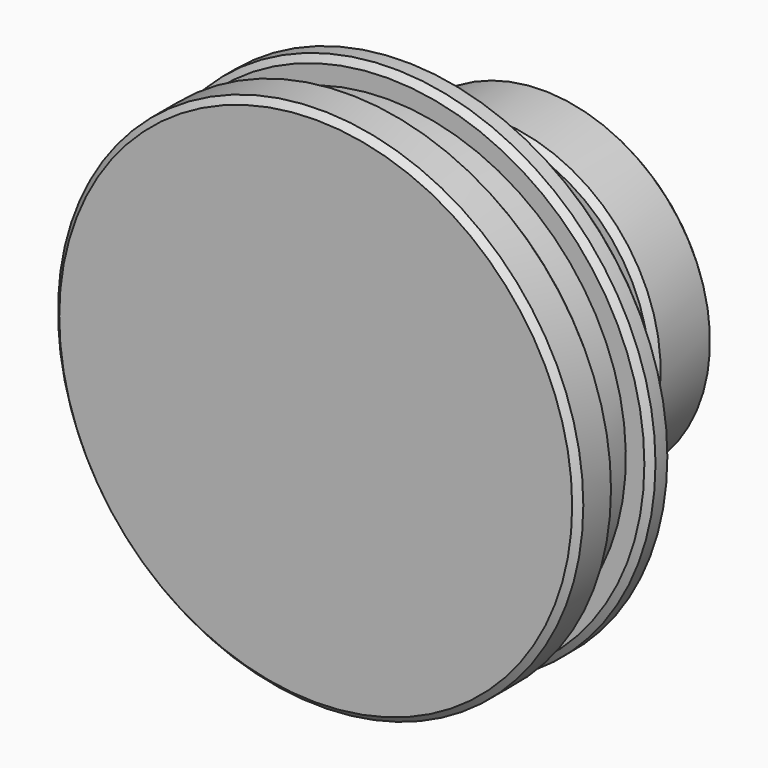
from build123d import *

# Parameters (mm, degrees)
F0_R     = 42.5
F1_DEPTH = 19
F2_W     = 7
F2_H     = 4
F4_R     = 30
F5_DEPTH = 16
F6_R     = 27
F7_DEPTH = 12


# Not quite as in the source:
# - a fillet or chamfer that OpenCascade refuses, or shapes differently, is made with other operations: its cross-section is extruded or revolved along the edge and cut away or added


with BuildPart() as f1:
    # F0 (on Front) → F1 (new body)
    with BuildSketch(Plane.XZ):
        Circle(F0_R)
    extrude(amount=F1_DEPTH)

    # F2 (on Right) → F3 (revolve, cut)
    with BuildSketch(Plane.YZ):
        with Locations((-7.9, 40.5)):
            Rectangle(F2_W, F2_H)
    revolve(axis=Axis((0, 0, 0), (0, 1, 0)), mode=Mode.SUBTRACT)

    # F4 (on face) → F5 (join)
    with BuildSketch(Plane(origin=(0, 0, 0), x_dir=(-1, 0, 0), z_dir=(0, 1, 0))):
        Circle(F4_R)
    extrude(amount=F5_DEPTH)

    # F6 (on face) → F7 (join)
    with BuildSketch(Plane(origin=(0, 16, 0), x_dir=(-1, 0, 0), z_dir=(0, 1, 0))):
        Circle(F6_R)
    extrude(amount=F7_DEPTH)

    # F8 (on Top) → F9 (revolve, cut)
    with BuildSketch(Plane.XY):
        Polygon((-30, 16), (-30, 0), (-28.6875, 7), (-18.6875, 7), (-18.6875, 16), align=None)
    revolve(axis=Axis((0, 23.2052635401, 0), (0, 1, 0)), mode=Mode.SUBTRACT)

    # F10: chamfer of 1 on 8 edges, made by hand

    # F10_s1 → F10_t2 (revolve, cut)
    with BuildSketch(Plane.XY):
        Polygon((42.5, -3.4), (41.5, -4.4), (42.5, -4.4), align=None)
    revolve(axis=Axis((0, -4.4, 0), (0, 1, 0)), mode=Mode.SUBTRACT)

    # F10_s3 → F10_t4 (revolve, cut)
    with BuildSketch(Plane.XY):
        Polygon((41.5, -11.4), (42.5, -12.4), (42.5, -11.4), align=None)
    revolve(axis=Axis((0, -11.4, 0), (0, 1, 0)), mode=Mode.SUBTRACT)

    # F10_s5 → F10_t6 (revolve, cut)
    with BuildSketch(Plane.XY):
        Polygon((42.5, -18), (41.5, -19), (42.5, -19), align=None)
    revolve(axis=Axis((0, -19, 0), (0, -1, 0)), mode=Mode.SUBTRACT)

    # F10_s7 → F10_t8 (revolve, cut)
    with BuildSketch(Plane.XY):
        Polygon((42.5, -1), (41.5, 0), (42.5, 0), align=None)
    revolve(axis=Axis((0, 0, 0), (0, -1, 0)), mode=Mode.SUBTRACT)

    # F10_s9 → F10_t10 (revolve, cut)
    with BuildSketch(Plane.XY):
        Polygon((-28.8404458997, 6.1842885351), (-27.8575737127, 7), (-28.6875, 7), align=None)
    revolve(axis=Axis((0, 7, 0), (0, 1, 0)), mode=Mode.SUBTRACT)

    # F10_s11 → F10_t12 (revolve, cut)
    with BuildSketch(Plane.XY):
        Polygon((-26, 16), (-27, 17), (-27, 16), align=None)
    revolve(axis=Axis((0, 16, 0), (0, 1, 0)), mode=Mode.SUBTRACT)

    # F10_s13 → F10_t14 (revolve, cut)
    with BuildSketch(Plane.XY):
        Polygon((-27, 27), (-26, 28), (-27, 28), align=None)
    revolve(axis=Axis((0, 28, 0), (0, 1, 0)), mode=Mode.SUBTRACT)


solid = f1.part
